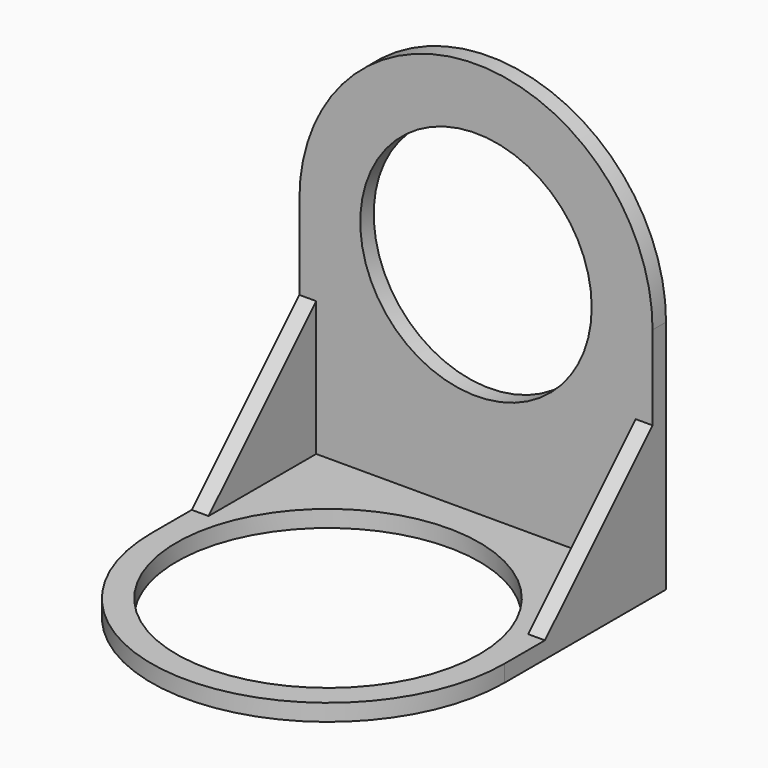
from build123d import *

# Parameters (mm, degrees)
F1_R     = 21.844
F2_DEPTH = 3.175
F3_R     = 28.575
F4_DEPTH = 3.175
F6_DEPTH = 3.175


# Not quite as in the source:
# - a variable given as a bare number and used for a length is read in inches; the dataset says mm whatever the document's units were


with BuildPart() as f2:
    # F1 (on Front) → F2 (new body)
    with BuildSketch(Plane.XZ):
        with BuildLine():
            Line((33.3375, 0), (33.3375, 44.45))
            ThreePointArc((33.3375, 44.45), (0, 77.7875), (-33.3375, 44.45))
            Line((-33.3375, 44.45), (-33.3375, 0))
            Line((-33.3375, 0), (33.3375, 0))
        make_face()
        with Locations((0, 44.45)):
            Circle(F1_R, mode=Mode.SUBTRACT)
    extrude(amount=F2_DEPTH)

    # F3 (on face) → F4 (join)
    with BuildSketch(Plane(origin=(0, 0, 0), x_dir=(1, 0, 0), z_dir=(0, 0, -1))):
        with BuildLine():
            Line((-33.3375, 38.1), (-33.3375, 3.175))
            Line((-33.3375, 3.175), (33.3375, 3.175))
            Line((33.3375, 3.175), (33.3375, 38.1))
            ThreePointArc((33.3375, 38.1), (0, 71.4375), (-33.3375, 38.1))
        make_face()
        with Locations((0, 38.1)):
            Circle(F3_R, mode=Mode.SUBTRACT)
    extrude(amount=-F4_DEPTH)

    # F5 (on face) → F6 (join)
    with BuildSketch(Plane.YZ.offset(33.3375)):
        Polygon((-3.175, 3.175), (-3.175, 28.575), (-28.575, 3.175), align=None)
    extrude(amount=-F6_DEPTH)

    # F7: F2 across plane


with BuildPart() as f2_1:
    add(f2.part)
    add(f2.part.mirror(Plane.YZ))


solid = f2_1.part
